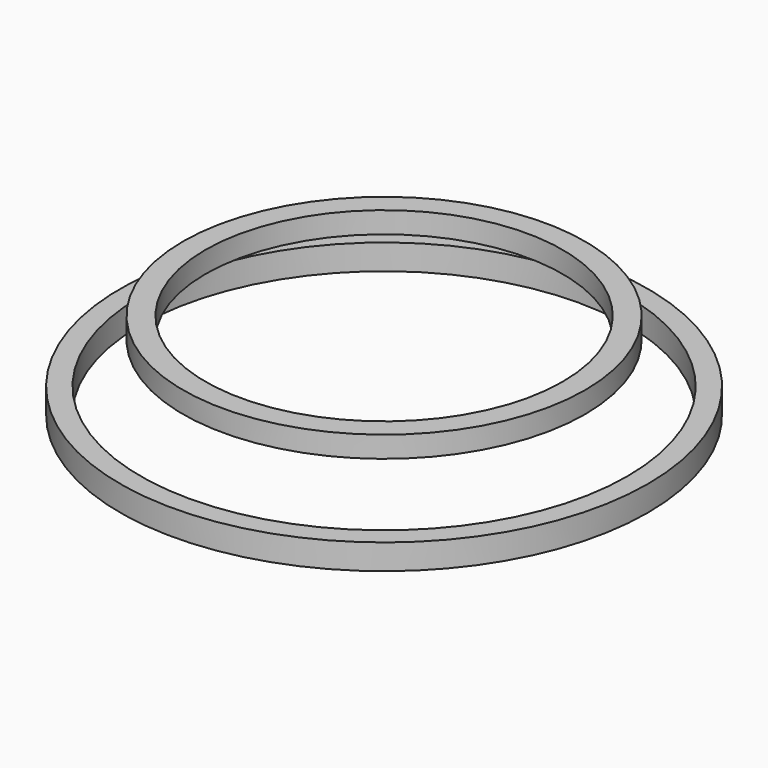
from build123d import *

# Parameters (mm, degrees)
F0_R     = 89.2252906984
F0_R_2   = 79.2252906984
F1_DEPTH = 9.4447415322
F3_R     = 117.0803624556
F3_R_2   = 107.9438435264
F4_DEPTH = 11.2299975008


# Not quite as in the source:
# - the program builds the solid bodies; features that only make, move or delete a surface that nothing else refers to are left out


with BuildPart() as f1:
    # F0 (on Top) → F1 (new body)
    with BuildSketch(Plane.XY):
        Circle(F0_R)
        Circle(F0_R_2, mode=Mode.SUBTRACT)
    extrude(amount=F1_DEPTH)


with BuildPart() as f4:
    # F3 (on offset) → F4 (new body)
    with BuildSketch(Plane.XY.offset(-29.3622110039)):
        Circle(F3_R)
        Circle(F3_R_2, mode=Mode.SUBTRACT)
    extrude(amount=F4_DEPTH)


solid = Compound([f1.part, f4.part])
